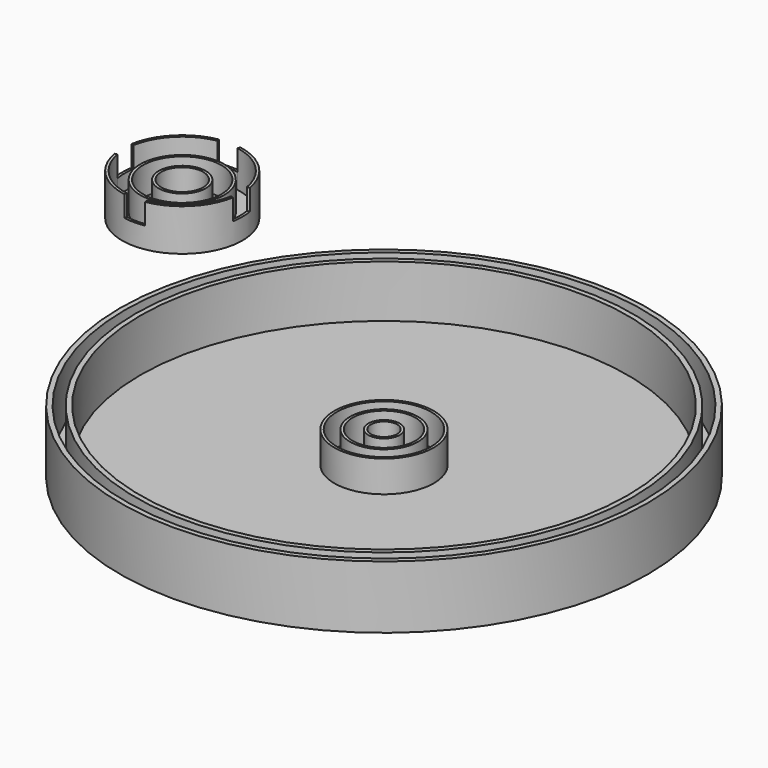
from build123d import *

# Parameters (mm, degrees)
F0_R      = 50.42
F0_R_2    = 49.46
F0_R_3    = 47.5
F0_R_4    = 46.54
F0_R_5    = 9.5
F0_R_6    = 9
F0_R_7    = 6.5
F0_R_8    = 6
F0_R_9    = 3
F0_R_10   = 2.5
F1_DEPTH  = 2
F2_DEPTH  = 12
F3_DEPTH  = 8
F4_R      = 8
F4_R_2    = 7.5
F4_R_3    = 4.5
F4_R_4    = 4
F5_DEPTH  = 1
F6_DEPTH  = 8
F7_DEPTH  = 8
F8_DEPTH  = 1.5
F9_DEPTH  = 1
F10_DEPTH = 4


with BuildPart() as f1:
    # F0 (on Top) → F1 (new body)
    with BuildSketch(Plane.XY):
        Circle(F0_R)
        Circle(F0_R_2, mode=Mode.SUBTRACT)
        Circle(F0_R_2)
        Circle(F0_R_3, mode=Mode.SUBTRACT)
        Circle(F0_R_3)
        Circle(F0_R_4, mode=Mode.SUBTRACT)
        Circle(F0_R_4)
        Circle(F0_R_5, mode=Mode.SUBTRACT)
        Circle(F0_R_5)
        Circle(F0_R_6, mode=Mode.SUBTRACT)
        Circle(F0_R_6)
        Circle(F0_R_7, mode=Mode.SUBTRACT)
        Circle(F0_R_7)
        Circle(F0_R_8, mode=Mode.SUBTRACT)
        Circle(F0_R_8)
        Circle(F0_R_9, mode=Mode.SUBTRACT)
        Circle(F0_R_9)
        Circle(F0_R_10, mode=Mode.SUBTRACT)
    extrude(amount=F1_DEPTH)

    # F0 (on Top) → F2 (join)
    with BuildSketch(Plane.XY):
        Circle(F0_R)
        Circle(F0_R_2, mode=Mode.SUBTRACT)
        Circle(F0_R_3)
        Circle(F0_R_4, mode=Mode.SUBTRACT)
    extrude(amount=F2_DEPTH)

    # F0 (on Top) → F3 (join)
    with BuildSketch(Plane.XY):
        Circle(F0_R_5)
        Circle(F0_R_6, mode=Mode.SUBTRACT)
        Circle(F0_R_7)
        Circle(F0_R_8, mode=Mode.SUBTRACT)
        Circle(F0_R_9)
        Circle(F0_R_10, mode=Mode.SUBTRACT)
    extrude(amount=F3_DEPTH)


with BuildPart() as f5:
    # F4 (on Top) → F5 (new body)
    with BuildSketch(Plane.XY):
        with BuildLine():
            ThreePointArc((-64.8501688035, 44.5327253536), (-66.1871253252, 46.4196205139), (-64.8501688035, 48.3065156742))
            ThreePointArc((-64.8501688035, 48.3065156742), (-67.9089507322, 54.197795107), (-73.8002301649, 57.2565770357))
            ThreePointArc((-73.8002301649, 57.2565770357), (-75.6871253252, 55.9196205139), (-77.5740204855, 57.2565770357))
            ThreePointArc((-77.5740204855, 57.2565770357), (-83.4652999183, 54.197795107), (-86.5240818469, 48.3065156742))
            ThreePointArc((-86.5240818469, 48.3065156742), (-85.5552419108, 47.5758888745), (-85.1871253252, 46.4196205139))
            ThreePointArc((-85.1871253252, 46.4196205139), (-85.5552419108, 45.2633521533), (-86.5240818469, 44.5327253536))
            ThreePointArc((-86.5240818469, 44.5327253536), (-83.4652999183, 38.6414459209), (-77.5740204855, 35.5826639922))
            ThreePointArc((-77.5740204855, 35.5826639922), (-75.6871253252, 36.9196205139), (-73.8002301649, 35.5826639922))
            ThreePointArc((-73.8002301649, 35.5826639922), (-67.9089507322, 38.6414459209), (-64.8501688035, 44.5327253536))
        make_face()
        with Locations((-75.6871253252, 46.4196205139)):
            Circle(F4_R, mode=Mode.SUBTRACT)
        with Locations((-75.6871253252, 46.4196205139)):
            Circle(F4_R)
        with Locations((-75.6871253252, 46.4196205139)):
            Circle(F4_R_2, mode=Mode.SUBTRACT)
        with Locations((-75.6871253252, 46.4196205139)):
            Circle(F4_R_2)
        with Locations((-75.6871253252, 46.4196205139)):
            Circle(F4_R_3, mode=Mode.SUBTRACT)
        with Locations((-75.6871253252, 46.4196205139)):
            Circle(F4_R_3)
        with Locations((-75.6871253252, 46.4196205139)):
            Circle(F4_R_4, mode=Mode.SUBTRACT)
        with Locations((-75.6871253252, 46.4196205139)):
            Circle(F4_R_4)
        with BuildLine():
            ThreePointArc((-73.8002301649, 57.2565770357), (-67.9089507322, 54.197795107), (-64.8501688035, 48.3065156742))
            ThreePointArc((-64.8501688035, 48.3065156742), (-64.6089169209, 48.374637611), (-64.3610383687, 48.4120447291))
            ThreePointArc((-64.3610383687, 48.4120447291), (-67.5553973416, 54.5513484976), (-73.69470111, 57.7457074704))
            ThreePointArc((-73.69470111, 57.7457074704), (-73.7321082281, 57.4978289182), (-73.8002301649, 57.2565770357))
        make_face()
        with BuildLine():
            ThreePointArc((-86.5240818469, 48.3065156742), (-83.4652999183, 54.197795107), (-77.5740204855, 57.2565770357))
            ThreePointArc((-77.5740204855, 57.2565770357), (-77.6421424223, 57.4978289182), (-77.6795495404, 57.7457074704))
            ThreePointArc((-77.6795495404, 57.7457074704), (-83.8188533088, 54.5513484976), (-87.0132122817, 48.4120447291))
            ThreePointArc((-87.0132122817, 48.4120447291), (-86.7653337295, 48.374637611), (-86.5240818469, 48.3065156742))
        make_face()
        with BuildLine():
            ThreePointArc((-77.6795495404, 35.0935335574), (-77.6421424223, 35.3414121096), (-77.5740204855, 35.5826639922))
            ThreePointArc((-77.5740204855, 35.5826639922), (-83.4652999183, 38.6414459209), (-86.5240818469, 44.5327253536))
            ThreePointArc((-86.5240818469, 44.5327253536), (-86.7653337295, 44.4646034168), (-87.0132122817, 44.4271962987))
            ThreePointArc((-87.0132122817, 44.4271962987), (-83.8188533088, 38.2878925303), (-77.6795495404, 35.0935335574))
        make_face()
        with BuildLine():
            ThreePointArc((-64.3610383687, 44.4271962987), (-64.6089169209, 44.4646034168), (-64.8501688035, 44.5327253536))
            ThreePointArc((-64.8501688035, 44.5327253536), (-67.9089507322, 38.6414459209), (-73.8002301649, 35.5826639922))
            ThreePointArc((-73.8002301649, 35.5826639922), (-73.7321082281, 35.3414121096), (-73.69470111, 35.0935335574))
            ThreePointArc((-73.69470111, 35.0935335574), (-67.5553973416, 38.2878925303), (-64.3610383687, 44.4271962987))
        make_face()
        with BuildLine():
            ThreePointArc((-77.5740204855, 57.2565770357), (-75.6871253252, 57.4196205139), (-73.8002301649, 57.2565770357))
            ThreePointArc((-73.8002301649, 57.2565770357), (-73.7321082281, 57.4978289182), (-73.69470111, 57.7457074704))
            ThreePointArc((-73.69470111, 57.7457074704), (-75.6871253252, 57.9196205139), (-77.6795495404, 57.7457074704))
            ThreePointArc((-77.6795495404, 57.7457074704), (-77.6421424223, 57.4978289182), (-77.5740204855, 57.2565770357))
        make_face()
        with BuildLine():
            ThreePointArc((-86.5240818469, 44.5327253536), (-86.6871253252, 46.4196205139), (-86.5240818469, 48.3065156742))
            ThreePointArc((-86.5240818469, 48.3065156742), (-86.7653337295, 48.374637611), (-87.0132122817, 48.4120447291))
            ThreePointArc((-87.0132122817, 48.4120447291), (-87.1871253252, 46.4196205139), (-87.0132122817, 44.4271962987))
            ThreePointArc((-87.0132122817, 44.4271962987), (-86.7653337295, 44.4646034168), (-86.5240818469, 44.5327253536))
        make_face()
        with BuildLine():
            ThreePointArc((-73.69470111, 35.0935335574), (-73.7321082281, 35.3414121096), (-73.8002301649, 35.5826639922))
            ThreePointArc((-73.8002301649, 35.5826639922), (-75.6871253252, 35.4196205139), (-77.5740204855, 35.5826639922))
            ThreePointArc((-77.5740204855, 35.5826639922), (-77.6421424223, 35.3414121096), (-77.6795495404, 35.0935335574))
            ThreePointArc((-77.6795495404, 35.0935335574), (-75.6871253252, 34.9196205139), (-73.69470111, 35.0935335574))
        make_face()
        with BuildLine():
            ThreePointArc((-64.8501688035, 48.3065156742), (-64.7279619963, 47.3665836232), (-64.6871253252, 46.4196205139))
            ThreePointArc((-64.6871253252, 46.4196205139), (-64.7279619963, 45.4726574046), (-64.8501688035, 44.5327253536))
            ThreePointArc((-64.8501688035, 44.5327253536), (-64.6089169209, 44.4646034168), (-64.3610383687, 44.4271962987))
            ThreePointArc((-64.3610383687, 44.4271962987), (-64.2306860878, 45.4196205139), (-64.1871253252, 46.4196205139))
            ThreePointArc((-64.1871253252, 46.4196205139), (-64.2306860878, 47.4196205139), (-64.3610383687, 48.4120447291))
            ThreePointArc((-64.3610383687, 48.4120447291), (-64.6089169209, 48.374637611), (-64.8501688035, 48.3065156742))
        make_face()
    extrude(amount=F5_DEPTH)

    # F4 (on Top) → F6 (join)
    with BuildSketch(Plane.XY):
        with BuildLine():
            ThreePointArc((-73.8002301649, 57.2565770357), (-67.9089507322, 54.197795107), (-64.8501688035, 48.3065156742))
            ThreePointArc((-64.8501688035, 48.3065156742), (-64.6089169209, 48.374637611), (-64.3610383687, 48.4120447291))
            ThreePointArc((-64.3610383687, 48.4120447291), (-67.5553973416, 54.5513484976), (-73.69470111, 57.7457074704))
            ThreePointArc((-73.69470111, 57.7457074704), (-73.7321082281, 57.4978289182), (-73.8002301649, 57.2565770357))
        make_face()
        with BuildLine():
            ThreePointArc((-77.5740204855, 57.2565770357), (-75.6871253252, 57.4196205139), (-73.8002301649, 57.2565770357))
            ThreePointArc((-73.8002301649, 57.2565770357), (-73.7321082281, 57.4978289182), (-73.69470111, 57.7457074704))
            ThreePointArc((-73.69470111, 57.7457074704), (-75.6871253252, 57.9196205139), (-77.6795495404, 57.7457074704))
            ThreePointArc((-77.6795495404, 57.7457074704), (-77.6421424223, 57.4978289182), (-77.5740204855, 57.2565770357))
        make_face()
        with BuildLine():
            ThreePointArc((-86.5240818469, 48.3065156742), (-83.4652999183, 54.197795107), (-77.5740204855, 57.2565770357))
            ThreePointArc((-77.5740204855, 57.2565770357), (-77.6421424223, 57.4978289182), (-77.6795495404, 57.7457074704))
            ThreePointArc((-77.6795495404, 57.7457074704), (-83.8188533088, 54.5513484976), (-87.0132122817, 48.4120447291))
            ThreePointArc((-87.0132122817, 48.4120447291), (-86.7653337295, 48.374637611), (-86.5240818469, 48.3065156742))
        make_face()
        with BuildLine():
            ThreePointArc((-86.5240818469, 44.5327253536), (-86.6871253252, 46.4196205139), (-86.5240818469, 48.3065156742))
            ThreePointArc((-86.5240818469, 48.3065156742), (-86.7653337295, 48.374637611), (-87.0132122817, 48.4120447291))
            ThreePointArc((-87.0132122817, 48.4120447291), (-87.1871253252, 46.4196205139), (-87.0132122817, 44.4271962987))
            ThreePointArc((-87.0132122817, 44.4271962987), (-86.7653337295, 44.4646034168), (-86.5240818469, 44.5327253536))
        make_face()
        with BuildLine():
            ThreePointArc((-77.6795495404, 35.0935335574), (-77.6421424223, 35.3414121096), (-77.5740204855, 35.5826639922))
            ThreePointArc((-77.5740204855, 35.5826639922), (-83.4652999183, 38.6414459209), (-86.5240818469, 44.5327253536))
            ThreePointArc((-86.5240818469, 44.5327253536), (-86.7653337295, 44.4646034168), (-87.0132122817, 44.4271962987))
            ThreePointArc((-87.0132122817, 44.4271962987), (-83.8188533088, 38.2878925303), (-77.6795495404, 35.0935335574))
        make_face()
        with BuildLine():
            ThreePointArc((-73.69470111, 35.0935335574), (-73.7321082281, 35.3414121096), (-73.8002301649, 35.5826639922))
            ThreePointArc((-73.8002301649, 35.5826639922), (-75.6871253252, 35.4196205139), (-77.5740204855, 35.5826639922))
            ThreePointArc((-77.5740204855, 35.5826639922), (-77.6421424223, 35.3414121096), (-77.6795495404, 35.0935335574))
            ThreePointArc((-77.6795495404, 35.0935335574), (-75.6871253252, 34.9196205139), (-73.69470111, 35.0935335574))
        make_face()
        with BuildLine():
            ThreePointArc((-64.3610383687, 44.4271962987), (-64.6089169209, 44.4646034168), (-64.8501688035, 44.5327253536))
            ThreePointArc((-64.8501688035, 44.5327253536), (-67.9089507322, 38.6414459209), (-73.8002301649, 35.5826639922))
            ThreePointArc((-73.8002301649, 35.5826639922), (-73.7321082281, 35.3414121096), (-73.69470111, 35.0935335574))
            ThreePointArc((-73.69470111, 35.0935335574), (-67.5553973416, 38.2878925303), (-64.3610383687, 44.4271962987))
        make_face()
        with BuildLine():
            ThreePointArc((-64.8501688035, 48.3065156742), (-64.7279619963, 47.3665836232), (-64.6871253252, 46.4196205139))
            ThreePointArc((-64.6871253252, 46.4196205139), (-64.7279619963, 45.4726574046), (-64.8501688035, 44.5327253536))
            ThreePointArc((-64.8501688035, 44.5327253536), (-64.6089169209, 44.4646034168), (-64.3610383687, 44.4271962987))
            ThreePointArc((-64.3610383687, 44.4271962987), (-64.2306860878, 45.4196205139), (-64.1871253252, 46.4196205139))
            ThreePointArc((-64.1871253252, 46.4196205139), (-64.2306860878, 47.4196205139), (-64.3610383687, 48.4120447291))
            ThreePointArc((-64.3610383687, 48.4120447291), (-64.6089169209, 48.374637611), (-64.8501688035, 48.3065156742))
        make_face()
        with Locations((-75.6871253252, 46.4196205139)):
            Circle(F4_R)
        with Locations((-75.6871253252, 46.4196205139)):
            Circle(F4_R_2, mode=Mode.SUBTRACT)
        with Locations((-75.6871253252, 46.4196205139)):
            Circle(F4_R_3)
        with Locations((-75.6871253252, 46.4196205139)):
            Circle(F4_R_4, mode=Mode.SUBTRACT)
    extrude(amount=F6_DEPTH)

    # F4 (on Top) → F7 (cut)
    with BuildSketch(Plane.XY):
        with BuildLine():
            ThreePointArc((-64.8501688035, 48.3065156742), (-64.7279619963, 47.3665836232), (-64.6871253252, 46.4196205139))
            ThreePointArc((-64.6871253252, 46.4196205139), (-64.7279619963, 45.4726574046), (-64.8501688035, 44.5327253536))
            ThreePointArc((-64.8501688035, 44.5327253536), (-64.6089169209, 44.4646034168), (-64.3610383687, 44.4271962987))
            ThreePointArc((-64.3610383687, 44.4271962987), (-64.2306860878, 45.4196205139), (-64.1871253252, 46.4196205139))
            ThreePointArc((-64.1871253252, 46.4196205139), (-64.2306860878, 47.4196205139), (-64.3610383687, 48.4120447291))
            ThreePointArc((-64.3610383687, 48.4120447291), (-64.6089169209, 48.374637611), (-64.8501688035, 48.3065156742))
        make_face()
        with BuildLine():
            ThreePointArc((-77.5740204855, 57.2565770357), (-75.6871253252, 57.4196205139), (-73.8002301649, 57.2565770357))
            ThreePointArc((-73.8002301649, 57.2565770357), (-73.7321082281, 57.4978289182), (-73.69470111, 57.7457074704))
            ThreePointArc((-73.69470111, 57.7457074704), (-75.6871253252, 57.9196205139), (-77.6795495404, 57.7457074704))
            ThreePointArc((-77.6795495404, 57.7457074704), (-77.6421424223, 57.4978289182), (-77.5740204855, 57.2565770357))
        make_face()
        with BuildLine():
            ThreePointArc((-73.69470111, 35.0935335574), (-73.7321082281, 35.3414121096), (-73.8002301649, 35.5826639922))
            ThreePointArc((-73.8002301649, 35.5826639922), (-75.6871253252, 35.4196205139), (-77.5740204855, 35.5826639922))
            ThreePointArc((-77.5740204855, 35.5826639922), (-77.6421424223, 35.3414121096), (-77.6795495404, 35.0935335574))
            ThreePointArc((-77.6795495404, 35.0935335574), (-75.6871253252, 34.9196205139), (-73.69470111, 35.0935335574))
        make_face()
        with BuildLine():
            ThreePointArc((-86.5240818469, 44.5327253536), (-86.6871253252, 46.4196205139), (-86.5240818469, 48.3065156742))
            ThreePointArc((-86.5240818469, 48.3065156742), (-86.7653337295, 48.374637611), (-87.0132122817, 48.4120447291))
            ThreePointArc((-87.0132122817, 48.4120447291), (-87.1871253252, 46.4196205139), (-87.0132122817, 44.4271962987))
            ThreePointArc((-87.0132122817, 44.4271962987), (-86.7653337295, 44.4646034168), (-86.5240818469, 44.5327253536))
        make_face()
    extrude(amount=F7_DEPTH, mode=Mode.SUBTRACT)

    # F8 (cut): faces of the model
    f8_faces = [f5.faces().sort_by_distance(p)[0] for p in [
        (-83.4608511552, 46.4196205139, 8),
        (-80.0598461046, 46.4196205139, 8),
    ]]
    extrude(f8_faces, amount=-F8_DEPTH, mode=Mode.SUBTRACT)

    # F4 (on Top) → F9 (join)
    with BuildSketch(Plane.XY):
        with BuildLine():
            ThreePointArc((-64.8501688035, 44.5327253536), (-64.7279619963, 45.4726574046), (-64.6871253252, 46.4196205139))
            ThreePointArc((-64.6871253252, 46.4196205139), (-64.7279619963, 47.3665836232), (-64.8501688035, 48.3065156742))
            ThreePointArc((-64.8501688035, 48.3065156742), (-66.1871253252, 46.4196205139), (-64.8501688035, 44.5327253536))
        make_face()
        with BuildLine():
            ThreePointArc((-64.8501688035, 48.3065156742), (-64.7279619963, 47.3665836232), (-64.6871253252, 46.4196205139))
            ThreePointArc((-64.6871253252, 46.4196205139), (-64.7279619963, 45.4726574046), (-64.8501688035, 44.5327253536))
            ThreePointArc((-64.8501688035, 44.5327253536), (-64.6089169209, 44.4646034168), (-64.3610383687, 44.4271962987))
            ThreePointArc((-64.3610383687, 44.4271962987), (-64.2306860878, 45.4196205139), (-64.1871253252, 46.4196205139))
            ThreePointArc((-64.1871253252, 46.4196205139), (-64.2306860878, 47.4196205139), (-64.3610383687, 48.4120447291))
            ThreePointArc((-64.3610383687, 48.4120447291), (-64.6089169209, 48.374637611), (-64.8501688035, 48.3065156742))
        make_face()
        with BuildLine():
            ThreePointArc((-77.5740204855, 57.2565770357), (-75.6871253252, 55.9196205139), (-73.8002301649, 57.2565770357))
            ThreePointArc((-73.8002301649, 57.2565770357), (-75.6871253252, 57.4196205139), (-77.5740204855, 57.2565770357))
        make_face()
        with BuildLine():
            ThreePointArc((-77.5740204855, 57.2565770357), (-75.6871253252, 57.4196205139), (-73.8002301649, 57.2565770357))
            ThreePointArc((-73.8002301649, 57.2565770357), (-73.7321082281, 57.4978289182), (-73.69470111, 57.7457074704))
            ThreePointArc((-73.69470111, 57.7457074704), (-75.6871253252, 57.9196205139), (-77.6795495404, 57.7457074704))
            ThreePointArc((-77.6795495404, 57.7457074704), (-77.6421424223, 57.4978289182), (-77.5740204855, 57.2565770357))
        make_face()
        with BuildLine():
            ThreePointArc((-73.69470111, 35.0935335574), (-73.7321082281, 35.3414121096), (-73.8002301649, 35.5826639922))
            ThreePointArc((-73.8002301649, 35.5826639922), (-75.6871253252, 35.4196205139), (-77.5740204855, 35.5826639922))
            ThreePointArc((-77.5740204855, 35.5826639922), (-77.6421424223, 35.3414121096), (-77.6795495404, 35.0935335574))
            ThreePointArc((-77.6795495404, 35.0935335574), (-75.6871253252, 34.9196205139), (-73.69470111, 35.0935335574))
        make_face()
        with BuildLine():
            ThreePointArc((-77.5740204855, 35.5826639922), (-75.6871253252, 35.4196205139), (-73.8002301649, 35.5826639922))
            ThreePointArc((-73.8002301649, 35.5826639922), (-75.6871253252, 36.9196205139), (-77.5740204855, 35.5826639922))
        make_face()
        with BuildLine():
            ThreePointArc((-85.1871253252, 46.4196205139), (-85.5552419108, 47.5758888745), (-86.5240818469, 48.3065156742))
            ThreePointArc((-86.5240818469, 48.3065156742), (-86.6871253252, 46.4196205139), (-86.5240818469, 44.5327253536))
            ThreePointArc((-86.5240818469, 44.5327253536), (-85.5552419108, 45.2633521533), (-85.1871253252, 46.4196205139))
        make_face()
        with BuildLine():
            ThreePointArc((-86.5240818469, 44.5327253536), (-86.6871253252, 46.4196205139), (-86.5240818469, 48.3065156742))
            ThreePointArc((-86.5240818469, 48.3065156742), (-86.7653337295, 48.374637611), (-87.0132122817, 48.4120447291))
            ThreePointArc((-87.0132122817, 48.4120447291), (-87.1871253252, 46.4196205139), (-87.0132122817, 44.4271962987))
            ThreePointArc((-87.0132122817, 44.4271962987), (-86.7653337295, 44.4646034168), (-86.5240818469, 44.5327253536))
        make_face()
    extrude(amount=F9_DEPTH)

    # F4 (on Top) → F10 (join)
    with BuildSketch(Plane.XY):
        with BuildLine():
            ThreePointArc((-64.8501688035, 48.3065156742), (-64.7279619963, 47.3665836232), (-64.6871253252, 46.4196205139))
            ThreePointArc((-64.6871253252, 46.4196205139), (-64.7279619963, 45.4726574046), (-64.8501688035, 44.5327253536))
            ThreePointArc((-64.8501688035, 44.5327253536), (-64.6089169209, 44.4646034168), (-64.3610383687, 44.4271962987))
            ThreePointArc((-64.3610383687, 44.4271962987), (-64.2306860878, 45.4196205139), (-64.1871253252, 46.4196205139))
            ThreePointArc((-64.1871253252, 46.4196205139), (-64.2306860878, 47.4196205139), (-64.3610383687, 48.4120447291))
            ThreePointArc((-64.3610383687, 48.4120447291), (-64.6089169209, 48.374637611), (-64.8501688035, 48.3065156742))
        make_face()
        with BuildLine():
            ThreePointArc((-77.5740204855, 57.2565770357), (-75.6871253252, 57.4196205139), (-73.8002301649, 57.2565770357))
            ThreePointArc((-73.8002301649, 57.2565770357), (-73.7321082281, 57.4978289182), (-73.69470111, 57.7457074704))
            ThreePointArc((-73.69470111, 57.7457074704), (-75.6871253252, 57.9196205139), (-77.6795495404, 57.7457074704))
            ThreePointArc((-77.6795495404, 57.7457074704), (-77.6421424223, 57.4978289182), (-77.5740204855, 57.2565770357))
        make_face()
        with BuildLine():
            ThreePointArc((-73.69470111, 35.0935335574), (-73.7321082281, 35.3414121096), (-73.8002301649, 35.5826639922))
            ThreePointArc((-73.8002301649, 35.5826639922), (-75.6871253252, 35.4196205139), (-77.5740204855, 35.5826639922))
            ThreePointArc((-77.5740204855, 35.5826639922), (-77.6421424223, 35.3414121096), (-77.6795495404, 35.0935335574))
            ThreePointArc((-77.6795495404, 35.0935335574), (-75.6871253252, 34.9196205139), (-73.69470111, 35.0935335574))
        make_face()
        with BuildLine():
            ThreePointArc((-86.5240818469, 44.5327253536), (-86.6871253252, 46.4196205139), (-86.5240818469, 48.3065156742))
            ThreePointArc((-86.5240818469, 48.3065156742), (-86.7653337295, 48.374637611), (-87.0132122817, 48.4120447291))
            ThreePointArc((-87.0132122817, 48.4120447291), (-87.1871253252, 46.4196205139), (-87.0132122817, 44.4271962987))
            ThreePointArc((-87.0132122817, 44.4271962987), (-86.7653337295, 44.4646034168), (-86.5240818469, 44.5327253536))
        make_face()
    extrude(amount=F10_DEPTH)


solid = Compound([f1.part, f5.part])
